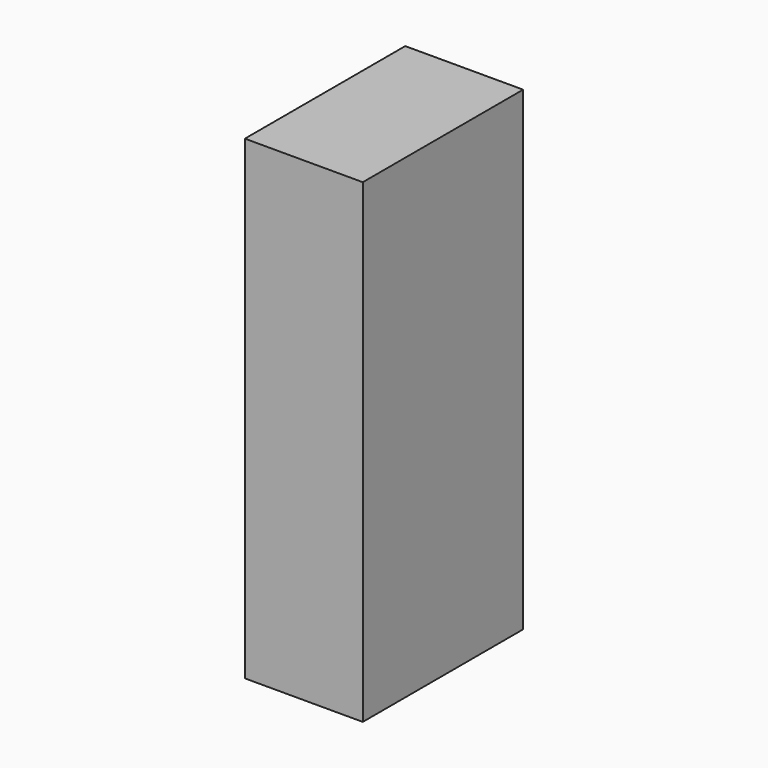
from build123d import *

# Parameters (mm, degrees)
F0_W     = 10
F0_H     = 40.3
F0_W_2   = 4.6593984449
F0_H_2   = 28.3
F1_DEPTH = 17
F2_DEPTH = 9


# Not quite as in the source:
# - a feature names something its author has since deleted; it is built from what else it names


with BuildPart() as f1:
    # F0 (on Front) → F1 (new body)
    with BuildSketch(Plane.XZ):
        with Locations((-25.2545091997, -60.7344553381)):
            Rectangle(F0_W, F0_H)
        with Locations((-25.3930282849, -60.7344553381)):
            Rectangle(F0_W_2, F0_H_2, mode=Mode.SUBTRACT)
        with Locations((-25.3930282849, -60.7344553381)):
            Rectangle(F0_W_2, F0_H_2)
    extrude(amount=F1_DEPTH)

    # F0 (on Front) → F2 (cut)
    with BuildSketch(Plane.XZ):
        with Locations((-25.3930282849, -60.7344553381)):
            Rectangle(F0_W_2, F0_H_2)
    extrude(amount=F2_DEPTH, mode=Mode.SUBTRACT)


solid = f1.part
